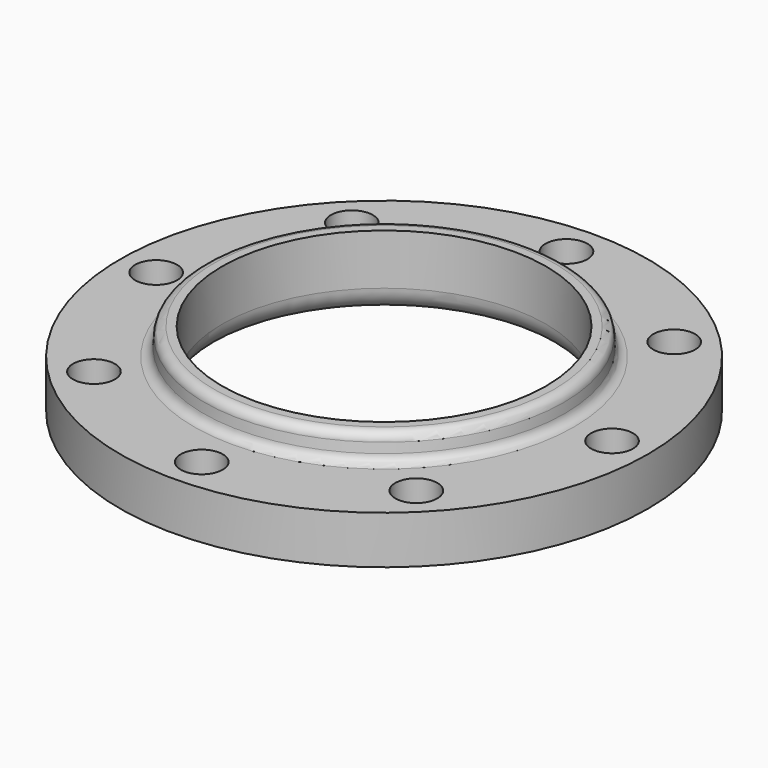
from build123d import *

# Parameters (mm, degrees)
F2_R     = 11.1
F3_DEPTH = 25.401


# Not quite as in the source:
# - a feature names something its author has since deleted; it is built from what else it names


with BuildPart() as f1:
    # F0 (on Front) → F1 (revolve)
    with BuildSketch(Plane.XZ):
        with BuildLine():
            ThreePointArc((85.75, 12.7), (89.4697438789, 3.7197438789), (98.45, 0))
            Line((98.45, 0), (139.7, 0))
            Line((139.7, 0), (139.7, 25.4))
            Line((139.7, 25.4), (100.5816558701, 25.4))
            ThreePointArc((100.5816558701, 25.4), (97.203704832, 26.7136133159), (95.6006823796, 29.9642212863))
            Line((95.6006823796, 29.9642212863), (95.1569785983, 35.0357787137))
            ThreePointArc((95.1569785983, 35.0357787137), (93.5539561459, 38.2863866841), (90.1760051078, 39.6))
            Line((90.1760051078, 39.6), (85.75, 39.6))
            Line((85.75, 39.6), (85.75, 12.7))
        make_face()
    revolve(axis=Axis((0, 0, 19.8), (0, 0, 1)))

    # F2 (on face) → F3 (cut, through all)
    with BuildSketch(Plane.XY.offset(25.4)):
        with Locations((0, 120.65)):
            Circle(F2_R)
        with Locations((-85.3124331502, 85.3124331502)):
            Circle(F2_R)
        with Locations((-120.65, 0)):
            Circle(F2_R)
        with Locations((-85.3124331502, -85.3124331502)):
            Circle(F2_R)
        with Locations((0, -120.65)):
            Circle(F2_R)
        with Locations((85.3124331502, -85.3124331502)):
            Circle(F2_R)
        with Locations((120.65, 0)):
            Circle(F2_R)
        with Locations((85.3124331502, 85.3124331502)):
            Circle(F2_R)
    extrude(amount=-F3_DEPTH, mode=Mode.SUBTRACT)


solid = f1.part
